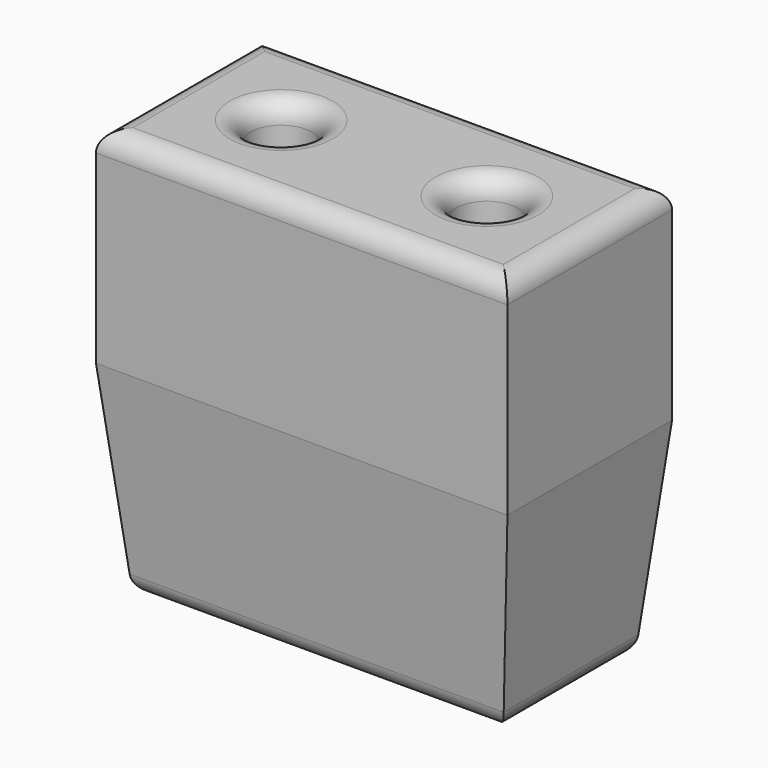
from build123d import *

# Parameters (mm, degrees)
F0_W        = 20
F0_H        = 10
F0_W_2      = 17.7
F0_H_2      = 7.5
F0_R        = 2.5
F0_R_2      = 1.5
F1_DEPTH    = 20
F2_DEPTH    = 5
F3_SIZE2    = 10
F3_SIZE     = 1
F4_T1_DEPTH = 22.5249378106
F4_T3_DEPTH = 12.5249378106
F4_T5_DEPTH = 25
F4_T7_DEPTH = 15


# Not quite as in the source:
# - a fillet or chamfer that OpenCascade refuses, or shapes differently, is made with other operations: its cross-section is extruded or revolved along the edge and cut away or added


with BuildPart() as f1:
    # F0 (on Top) → F1 (new body)
    with BuildSketch(Plane.XY):
        Rectangle(F0_W, F0_H)
        Rectangle(F0_W_2, F0_H_2, mode=Mode.SUBTRACT)
        Rectangle(F0_W_2, F0_H_2)
        with Locations((-5, 0)):
            Circle(F0_R, mode=Mode.SUBTRACT)
        with Locations((5, 0)):
            Circle(F0_R, mode=Mode.SUBTRACT)
        with Locations((5, 0)):
            Circle(F0_R)
        with Locations((5, 0)):
            Circle(F0_R_2, mode=Mode.SUBTRACT)
        with Locations((-5, 0)):
            Circle(F0_R)
        with Locations((-5, 0)):
            Circle(F0_R_2, mode=Mode.SUBTRACT)
    extrude(amount=F1_DEPTH)

    # F0 (on Top) → F2 (cut)
    with BuildSketch(Plane.XY):
        with Locations((-5, 0)):
            Circle(F0_R)
        with Locations((-5, 0)):
            Circle(F0_R_2, mode=Mode.SUBTRACT)
        with Locations((5, 0)):
            Circle(F0_R)
        with Locations((5, 0)):
            Circle(F0_R_2, mode=Mode.SUBTRACT)
    extrude(amount=F2_DEPTH, mode=Mode.SUBTRACT)

    # F3
    f3_edges = [f1.edges().sort_by_distance(p)[0] for p in [
        (0, -5, 0),
        (-10, 0, 0),
        (0, 5, 0),
        (10, 0, 0),
    ]]
    f3_side = f1.faces().sort_by_distance((0, 0, 0))[0]
    chamfer(f3_edges, length=F3_SIZE, length2=F3_SIZE2, reference=f3_side)

    # F4: fillet of radius 1 on 12 edges, made by hand

    # F4_s2 → F4_t1 (cut)
    with BuildSketch(Plane.YZ.offset(-11.2624689053)):
        with BuildLine():
            ThreePointArc((-3.0950124379, 0), (-3.7660177586, 0.2585474664), (-4.0900496281, 0.900496281))
            Line((-4.0900496281, 0.900496281), (-4, 0))
            Line((-4, 0), (-3.0950124379, 0))
        make_face()
        with BuildLine():
            ThreePointArc((4.0900496281, 0.900496281), (3.7660177586, 0.2585474664), (3.0950124379, 0))
            Line((3.0950124379, 0), (4, 0))
            Line((4, 0), (4.0900496281, 0.900496281))
        make_face()
    extrude(amount=F4_T1_DEPTH, mode=Mode.SUBTRACT)

    # F4_s4 → F4_t3 (cut)
    with BuildSketch(Plane.XZ.offset(-6.2624689053)):
        with BuildLine():
            ThreePointArc((-8.0950124379, 0), (-8.7660177586, 0.2585474664), (-9.0900496281, 0.900496281))
            Line((-9.0900496281, 0.900496281), (-9, 0))
            Line((-9, 0), (-8.0950124379, 0))
        make_face()
        with BuildLine():
            ThreePointArc((9.0900496281, 0.900496281), (8.7660177586, 0.2585474664), (8.0950124379, 0))
            Line((8.0950124379, 0), (9, 0))
            Line((9, 0), (9.0900496281, 0.900496281))
        make_face()
    extrude(amount=F4_T3_DEPTH, mode=Mode.SUBTRACT)

    # F4_s6 → F4_t5 (cut)
    with BuildSketch(Plane.YZ.offset(-12.5)):
        with BuildLine():
            ThreePointArc((-4, 20), (-4.7071067812, 19.7071067812), (-5, 19))
            Line((-5, 19), (-5, 20))
            Line((-5, 20), (-4, 20))
        make_face()
        with BuildLine():
            ThreePointArc((5, 19), (4.7071067812, 19.7071067812), (4, 20))
            Line((4, 20), (5, 20))
            Line((5, 20), (5, 19))
        make_face()
    extrude(amount=F4_T5_DEPTH, mode=Mode.SUBTRACT)

    # F4_s8 → F4_t7 (cut)
    with BuildSketch(Plane.XZ.offset(-7.5)):
        with BuildLine():
            ThreePointArc((10, 19), (9.7071067812, 19.7071067812), (9, 20))
            Line((9, 20), (10, 20))
            Line((10, 20), (10, 19))
        make_face()
        with BuildLine():
            ThreePointArc((-9, 20), (-9.7071067812, 19.7071067812), (-10, 19))
            Line((-10, 19), (-10, 20))
            Line((-10, 20), (-9, 20))
        make_face()
    extrude(amount=F4_T7_DEPTH, mode=Mode.SUBTRACT)

    # F4_s9 → F4_t10 (revolve, cut)
    with BuildSketch(Plane.XZ):
        with BuildLine():
            ThreePointArc((7.5, 20), (6.7928932188, 19.7071067812), (6.5, 19))
            Line((6.5, 19), (6.5, 20))
            Line((6.5, 20), (7.5, 20))
        make_face()
    revolve(axis=Axis((5, 0, 20), (0, 0, 1)), mode=Mode.SUBTRACT)

    # F4_s11 → F4_t12 (revolve, cut)
    with BuildSketch(Plane.XZ):
        with BuildLine():
            ThreePointArc((-2.5, 20), (-3.2071067812, 19.7071067812), (-3.5, 19))
            Line((-3.5, 19), (-3.5, 20))
            Line((-3.5, 20), (-2.5, 20))
        make_face()
    revolve(axis=Axis((-5, 0, 20), (0, 0, 1)), mode=Mode.SUBTRACT)

    # F4_s13 → F4_t14 (revolve, cut)
    with BuildSketch(Plane.XZ):
        with BuildLine():
            ThreePointArc((8.5, 0), (7.7928932188, 0.2928932188), (7.5, 1))
            Line((7.5, 1), (7.5, 0))
            Line((7.5, 0), (8.5, 0))
        make_face()
    revolve(axis=Axis((5, 0, 0), (0, 0, 1)), mode=Mode.SUBTRACT)

    # F4_s15 → F4_t16 (revolve, cut)
    with BuildSketch(Plane.XZ):
        with BuildLine():
            ThreePointArc((-1.5, 0), (-2.2071067812, 0.2928932188), (-2.5, 1))
            Line((-2.5, 1), (-2.5, 0))
            Line((-2.5, 0), (-1.5, 0))
        make_face()
    revolve(axis=Axis((-5, 0, 0), (0, 0, 1)), mode=Mode.SUBTRACT)


solid = f1.part
